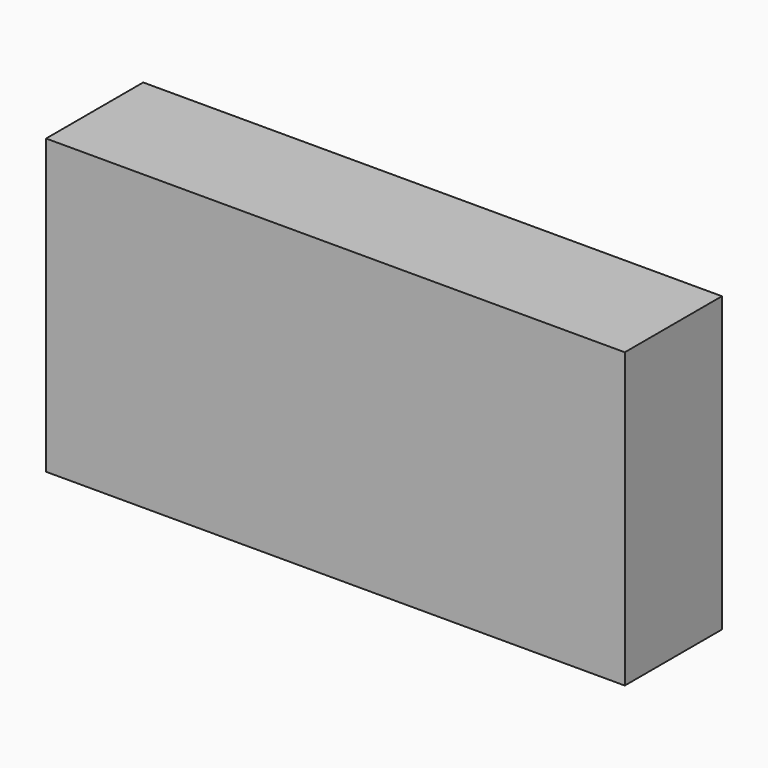
from build123d import *

# Parameters (mm, degrees)
F0_W     = 121.0717409849
F0_H     = 61.3841339946
F1_DEPTH = 25.4


# Not quite as in the source:
# - the program builds the solid bodies; features that only make, move or delete a surface that nothing else refers to are left out


with BuildPart() as f1:
    # F0 (on Front) → F1 (new body)
    with BuildSketch(Plane.XZ):
        with Locations((-45.0499504805, 6.4310319722)):
            Rectangle(F0_W, F0_H)
    extrude(amount=F1_DEPTH)


solid = f1.part
